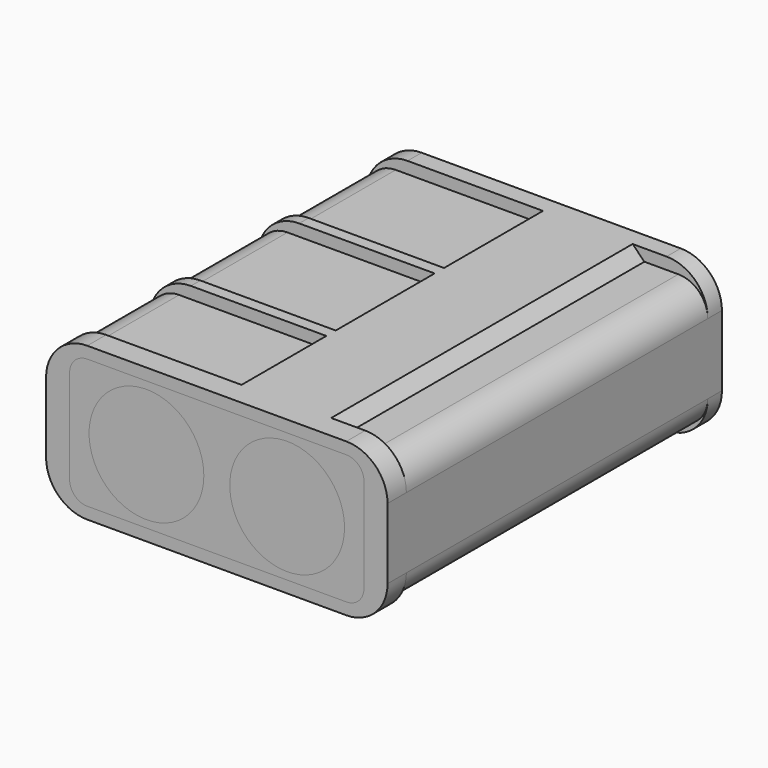
from build123d import *

# Parameters (mm, degrees)
F1_START      = 65
F0_W          = 50
F0_H          = 22
F0_R          = 9.75
F1_DEPTH      = 6
F2_R          = 3
F3_W          = 58
F3_H          = 26
F4_DEPTH      = 71
F5_DEPTH      = 6
F6_R          = 7
F8_START      = -11
F7_W          = 50
F7_H          = 21
F7_H_2        = 18
F7_W_2        = 22
F7_H_3        = 64
F8_DEPTH      = 17.9
F9_START      = 11
F9_DEPTH      = 6.8
F10_R         = 4.99999
F11_T4_DEPTH  = 46.7168298797
F11_T10_DEPTH = 21
F11_T15_DEPTH = 46.7168298797
F11_T21_DEPTH = 21
F11_T26_DEPTH = 46.7168298797
F11_T32_DEPTH = 18
F11_T37_DEPTH = 43.7168298797
F11_T43_DEPTH = 64
F11_T48_DEPTH = 46.7168298797
F11_T54_DEPTH = 21
F11_T59_DEPTH = 46.7168298797
F11_T65_DEPTH = 21
F11_T70_DEPTH = 46.7168298797
F11_T76_DEPTH = 18
F11_T81_DEPTH = 43.7168298797
F11_T87_DEPTH = 64


# Not quite as in the source:
# - a fillet or chamfer that OpenCascade refuses, or shapes differently, is made with other operations: its cross-section is extruded or revolved along the edge and cut away or added
# - a fillet or chamfer is up to 0.001 mm smaller than in the source, because OpenCascade refuses the exact size


with BuildPart() as f1:
    # F0 (on Front) → F1 (new body)
    with BuildSketch(Plane.XZ.offset(F1_START)):
        Rectangle(F0_W, F0_H)
        with Locations((-11.95, 0)):
            Circle(F0_R, mode=Mode.SUBTRACT)
        with Locations((11.95, 0)):
            Circle(F0_R, mode=Mode.SUBTRACT)
    extrude(amount=F1_DEPTH)

    # F2
    f2_edges = [f1.edges().sort_by_distance(p)[0] for p in [
        (25, -68, 11),
        (25, -68, -11),
        (-25, -68, 11),
        (-25, -68, -11),
    ]]
    fillet(f2_edges, radius=F2_R)


with BuildPart() as f4:
    # F3 (on Front) → F4 (new body)
    with BuildSketch(Plane.XZ):
        Rectangle(F3_W, F3_H)
    extrude(amount=F4_DEPTH)

    # F5 (cut): a face of the model
    f5_faces = [f1.part.faces().sort_by_distance(p)[0] for p in [
        (0, -71, 0),
    ]]
    extrude(f5_faces, amount=-F5_DEPTH, mode=Mode.SUBTRACT)

    # F6
    f6_edges = [f4.edges().sort_by_distance(p)[0] for p in [
        (-29, -35.5, 13),
        (-29, -35.5, -13),
        (29, -35.5, 13),
        (29, -35.5, -13),
    ]]
    fillet(f6_edges, radius=F6_R)

    # F7 (on Top) → F8 (cut)
    with BuildSketch(Plane.XY.offset(F8_START)):
        with Locations((-29, -13.5)):
            Rectangle(F7_W, F7_H)
        with Locations((-29, -36.5)):
            Rectangle(F7_W, F7_H)
        with Locations((-29, -58)):
            Rectangle(F7_W, F7_H_2)
        with Locations((32.2295585051, -35)):
            Rectangle(F7_W_2, F7_H_3)
    extrude(amount=-F8_DEPTH, mode=Mode.SUBTRACT)

    # F7 (on Top) → F9 (cut)
    with BuildSketch(Plane.XY.offset(F9_START)):
        with Locations((-29, -13.5)):
            Rectangle(F7_W, F7_H)
        with Locations((-29, -36.5)):
            Rectangle(F7_W, F7_H)
        with Locations((-29, -58)):
            Rectangle(F7_W, F7_H_2)
        with Locations((32.2295585051, -35)):
            Rectangle(F7_W_2, F7_H_3)
    extrude(amount=F9_DEPTH, mode=Mode.SUBTRACT)

    # F10 (radius 5 in the source; OpenCascade refuses exactly that, so slightly less here)
    f10_edges = [f4.edges().sort_by_distance(p)[0] for p in [
        (-26.898979, -36.5, 11),
        (-26.898979, -13.5, 11),
        (-26.898979, -58, 11),
        (26.898979, -35, 11),
        (-26.898979, -13.5, -11),
        (-26.898979, -36.5, -11),
        (-26.898979, -58, -11),
        (26.898979, -35, -11),
    ]]
    fillet(f10_edges, radius=F10_R)

    # F11: chamfer of 5 on 8 edges, made by hand


with BuildPart() as f11_tool2:
    # F11_s3 → F11_t4 (new body)
    with BuildSketch(Plane.XZ.offset(36.8584149398)):
        Polygon((1, 13), (-4, 8), (-4, 13), align=None)
    extrude(amount=-F11_T4_DEPTH)

    split(bisect_by=Plane.XZ.offset(26), keep=Keep.TOP)

    split(bisect_by=Plane.XY.offset(11), keep=Keep.TOP)


with BuildPart() as f4_1:
    add(f4.part)

    # F11_t1: cut F11_tool2
    add(f11_tool2.part, mode=Mode.SUBTRACT)


with BuildPart() as f11_tool8:
    # F11_s9 → F11_t10 (new body)
    with BuildSketch(Plane.XZ.offset(24)):
        Polygon((1, 13), (-4, 8), (-4, 13), align=None)
    extrude(amount=-F11_T10_DEPTH)

    split(bisect_by=Plane.XY.offset(11), keep=Keep.TOP)


with BuildPart() as f4_2:
    add(f4_1.part)

    # F11_t7: cut F11_tool8
    add(f11_tool8.part, mode=Mode.SUBTRACT)


with BuildPart() as f11_tool13:
    # F11_s14 → F11_t15 (new body)
    with BuildSketch(Plane.XZ.offset(59.8584149398)):
        Polygon((1, 13), (-4, 8), (-4, 13), align=None)
    extrude(amount=-F11_T15_DEPTH)

    split(bisect_by=Plane.XZ.offset(49), keep=Keep.TOP)

    split(bisect_by=Plane.XY.offset(11), keep=Keep.TOP)


with BuildPart() as f4_3:
    add(f4_2.part)

    # F11_t12: cut F11_tool13
    add(f11_tool13.part, mode=Mode.SUBTRACT)


with BuildPart() as f11_tool19:
    # F11_s20 → F11_t21 (new body)
    with BuildSketch(Plane.XZ.offset(47)):
        Polygon((1, 13), (-4, 8), (-4, 13), align=None)
    extrude(amount=-F11_T21_DEPTH)

    split(bisect_by=Plane.XY.offset(11), keep=Keep.TOP)


with BuildPart() as f4_4:
    add(f4_3.part)

    # F11_t18: cut F11_tool19
    add(f11_tool19.part, mode=Mode.SUBTRACT)


with BuildPart() as f11_tool24:
    # F11_s25 → F11_t26 (new body)
    with BuildSketch(Plane.XZ.offset(59.8584149398)):
        Polygon((1, 13), (-4, 8), (-4, 13), align=None)
    extrude(amount=-F11_T26_DEPTH)

    split(bisect_by=Plane.XZ.offset(24), keep=Keep.BOTTOM)

    split(bisect_by=Plane.XY.offset(11), keep=Keep.TOP)


with BuildPart() as f4_5:
    add(f4_4.part)

    # F11_t23: cut F11_tool24
    add(f11_tool24.part, mode=Mode.SUBTRACT)


with BuildPart() as f11_tool30:
    # F11_s31 → F11_t32 (new body)
    with BuildSketch(Plane.XZ.offset(67)):
        Polygon((1, 13), (-4, 8), (-4, 13), align=None)
    extrude(amount=-F11_T32_DEPTH)

    split(bisect_by=Plane.XY.offset(11), keep=Keep.TOP)


with BuildPart() as f4_6:
    add(f4_5.part)

    # F11_t29: cut F11_tool30
    add(f11_tool30.part, mode=Mode.SUBTRACT)


with BuildPart() as f11_tool35:
    # F11_s36 → F11_t37 (new body)
    with BuildSketch(Plane.XZ.offset(79.8584149398)):
        Polygon((1, 13), (-4, 8), (-4, 13), align=None)
    extrude(amount=-F11_T37_DEPTH)

    split(bisect_by=Plane.XZ.offset(47), keep=Keep.BOTTOM)

    split(bisect_by=Plane.XY.offset(11), keep=Keep.TOP)


with BuildPart() as f4_7:
    add(f4_6.part)

    # F11_t34: cut F11_tool35
    add(f11_tool35.part, mode=Mode.SUBTRACT)


with BuildPart() as f11_tool41:
    # F11_s42 → F11_t43 (new body)
    with BuildSketch(Plane.XZ.offset(3)):
        Polygon((16.2295585051, 13), (21.2295585051, 8), (21.2295585051, 13), align=None)
    extrude(amount=F11_T43_DEPTH)

    split(bisect_by=Plane.XY.offset(11), keep=Keep.TOP)


with BuildPart() as f4_8:
    add(f4_7.part)

    # F11_t40: cut F11_tool41
    add(f11_tool41.part, mode=Mode.SUBTRACT)


with BuildPart() as f11_tool46:
    # F11_s47 → F11_t48 (new body)
    with BuildSketch(Plane.XZ.offset(36.8584149398)):
        Polygon((1, -13), (-4, -8), (-4, -13), align=None)
    extrude(amount=-F11_T48_DEPTH)

    split(bisect_by=Plane.XZ.offset(26), keep=Keep.TOP)

    split(bisect_by=Plane.XY.offset(-11), keep=Keep.BOTTOM)


with BuildPart() as f4_9:
    add(f4_8.part)

    # F11_t45: cut F11_tool46
    add(f11_tool46.part, mode=Mode.SUBTRACT)


with BuildPart() as f11_tool52:
    # F11_s53 → F11_t54 (new body)
    with BuildSketch(Plane.XZ.offset(24)):
        Polygon((1, -13), (-4, -8), (-4, -13), align=None)
    extrude(amount=-F11_T54_DEPTH)

    split(bisect_by=Plane.XY.offset(-11), keep=Keep.BOTTOM)


with BuildPart() as f4_10:
    add(f4_9.part)

    # F11_t51: cut F11_tool52
    add(f11_tool52.part, mode=Mode.SUBTRACT)


with BuildPart() as f11_tool57:
    # F11_s58 → F11_t59 (new body)
    with BuildSketch(Plane.XZ.offset(59.8584149398)):
        Polygon((1, -13), (-4, -8), (-4, -13), align=None)
    extrude(amount=-F11_T59_DEPTH)

    split(bisect_by=Plane.XZ.offset(49), keep=Keep.TOP)

    split(bisect_by=Plane.XY.offset(-11), keep=Keep.BOTTOM)


with BuildPart() as f4_11:
    add(f4_10.part)

    # F11_t56: cut F11_tool57
    add(f11_tool57.part, mode=Mode.SUBTRACT)


with BuildPart() as f11_tool63:
    # F11_s64 → F11_t65 (new body)
    with BuildSketch(Plane.XZ.offset(47)):
        Polygon((1, -13), (-4, -8), (-4, -13), align=None)
    extrude(amount=-F11_T65_DEPTH)

    split(bisect_by=Plane.XY.offset(-11), keep=Keep.BOTTOM)


with BuildPart() as f4_12:
    add(f4_11.part)

    # F11_t62: cut F11_tool63
    add(f11_tool63.part, mode=Mode.SUBTRACT)


with BuildPart() as f11_tool68:
    # F11_s69 → F11_t70 (new body)
    with BuildSketch(Plane.XZ.offset(59.8584149398)):
        Polygon((1, -13), (-4, -8), (-4, -13), align=None)
    extrude(amount=-F11_T70_DEPTH)

    split(bisect_by=Plane.XZ.offset(24), keep=Keep.BOTTOM)

    split(bisect_by=Plane.XY.offset(-11), keep=Keep.BOTTOM)


with BuildPart() as f4_13:
    add(f4_12.part)

    # F11_t67: cut F11_tool68
    add(f11_tool68.part, mode=Mode.SUBTRACT)


with BuildPart() as f11_tool74:
    # F11_s75 → F11_t76 (new body)
    with BuildSketch(Plane.XZ.offset(67)):
        Polygon((1, -13), (-4, -8), (-4, -13), align=None)
    extrude(amount=-F11_T76_DEPTH)

    split(bisect_by=Plane.XY.offset(-11), keep=Keep.BOTTOM)


with BuildPart() as f4_14:
    add(f4_13.part)

    # F11_t73: cut F11_tool74
    add(f11_tool74.part, mode=Mode.SUBTRACT)


with BuildPart() as f11_tool79:
    # F11_s80 → F11_t81 (new body)
    with BuildSketch(Plane.XZ.offset(79.8584149398)):
        Polygon((1, -13), (-4, -8), (-4, -13), align=None)
    extrude(amount=-F11_T81_DEPTH)

    split(bisect_by=Plane.XZ.offset(47), keep=Keep.BOTTOM)

    split(bisect_by=Plane.XY.offset(-11), keep=Keep.BOTTOM)


with BuildPart() as f4_15:
    add(f4_14.part)

    # F11_t78: cut F11_tool79
    add(f11_tool79.part, mode=Mode.SUBTRACT)


with BuildPart() as f11_tool85:
    # F11_s86 → F11_t87 (new body)
    with BuildSketch(Plane.XZ.offset(3)):
        Polygon((16.2295585051, -13), (21.2295585051, -8), (21.2295585051, -13), align=None)
    extrude(amount=F11_T87_DEPTH)

    split(bisect_by=Plane.XY.offset(-11), keep=Keep.BOTTOM)


with BuildPart() as f4_16:
    add(f4_15.part)

    # F11_t84: cut F11_tool85
    add(f11_tool85.part, mode=Mode.SUBTRACT)


solid = Compound([f1.part, f4_16.part])
